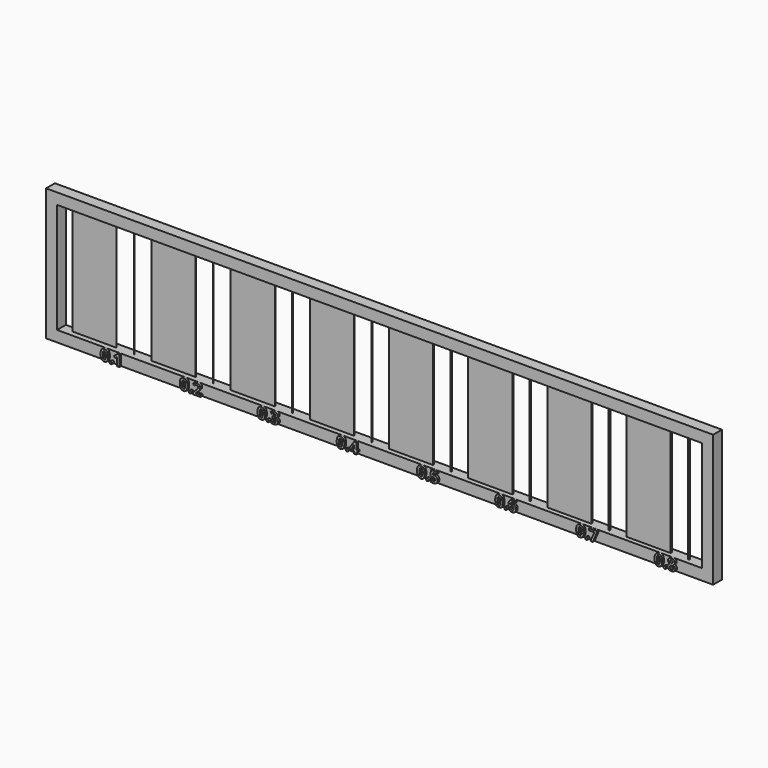
from build123d import *

# Parameters (mm, degrees)
F0_W          = 20
F0_H          = 0.1
F1_DEPTH      = 50
F0_H_2        = 0.2
F0_H_3        = 0.5
F0_H_4        = 0.6
F0_H_5        = 0.7
F0_H_6        = 0.8
F0_H_7        = 0.3
F0_H_8        = 0.4
F0_R          = 0.05
F0_R_2        = 0.1
F0_R_3        = 0.15
F0_R_4        = 0.2
F0_R_5        = 0.25
F0_R_6        = 0.3
F0_R_7        = 0.35
F0_R_8        = 0.4
F2_W          = 303
F2_H          = 60
F2_W_2        = 293
F2_H_2        = 50
F3_DEPTH      = 2.5
F3_DEPTH_BACK = 2.5
F4_TEXT_SIZE  = 6.9444444444
F5_DEPTH      = 1


# Not quite as in the source:
# - Text() gives the source's letters only with a copy of the font that has no kerning and outlines rounded to 1/6400 em; it was checked with that copy


with BuildPart() as f1:
    # F0 (on Top) → F1 (new body)
    with BuildSketch(Plane.XY):
        with Locations((-84.2978805304, 0)):
            Rectangle(F0_W, F0_H)
    extrude(amount=F1_DEPTH)


with BuildPart() as f1b:
    # F0 (on Top) → F1, piece 2 (new body)
    with BuildSketch(Plane.XY):
        with Locations((-48.2978805304, 0)):
            Rectangle(F0_W, F0_H_2)
    extrude(amount=F1_DEPTH)


with BuildPart() as f1c:
    # F0 (on Top) → F1, piece 3 (new body)
    with BuildSketch(Plane.XY):
        with Locations((59.7021194696, 0)):
            Rectangle(F0_W, F0_H_3)
    extrude(amount=F1_DEPTH)


with BuildPart() as f1d:
    # F0 (on Top) → F1, piece 4 (new body)
    with BuildSketch(Plane.XY):
        with Locations((95.7021194696, 0)):
            Rectangle(F0_W, F0_H_4)
    extrude(amount=F1_DEPTH)


with BuildPart() as f1e:
    # F0 (on Top) → F1, piece 5 (new body)
    with BuildSketch(Plane.XY):
        with Locations((131.7021194696, 0)):
            Rectangle(F0_W, F0_H_5)
    extrude(amount=F1_DEPTH)


with BuildPart() as f1f:
    # F0 (on Top) → F1, piece 6 (new body)
    with BuildSketch(Plane.XY):
        with Locations((167.7021194696, 0)):
            Rectangle(F0_W, F0_H_6)
    extrude(amount=F1_DEPTH)


with BuildPart() as f1g:
    # F0 (on Top) → F1, piece 7 (new body)
    with BuildSketch(Plane.XY):
        with Locations((-12.2978805304, 0)):
            Rectangle(F0_W, F0_H_7)
    extrude(amount=F1_DEPTH)


with BuildPart() as f1h:
    # F0 (on Top) → F1, piece 8 (new body)
    with BuildSketch(Plane.XY):
        with Locations((23.7021194696, 0)):
            Rectangle(F0_W, F0_H_8)
    extrude(amount=F1_DEPTH)


with BuildPart() as f1i:
    # F0 (on Top) → F1, piece 9 (new body)
    with BuildSketch(Plane.XY):
        with Locations((-66.2978805304, 0)):
            Circle(F0_R)
    extrude(amount=F1_DEPTH)


with BuildPart() as f1j:
    # F0 (on Top) → F1, piece 10 (new body)
    with BuildSketch(Plane.XY):
        with Locations((-30.2978805304, 0)):
            Circle(F0_R_2)
    extrude(amount=F1_DEPTH)


with BuildPart() as f1k:
    # F0 (on Top) → F1, piece 11 (new body)
    with BuildSketch(Plane.XY):
        with Locations((5.7021194696, 0)):
            Circle(F0_R_3)
    extrude(amount=F1_DEPTH)


with BuildPart() as f1l:
    # F0 (on Top) → F1, piece 12 (new body)
    with BuildSketch(Plane.XY):
        with Locations((41.7021194696, 0)):
            Circle(F0_R_4)
    extrude(amount=F1_DEPTH)


with BuildPart() as f1m:
    # F0 (on Top) → F1, piece 13 (new body)
    with BuildSketch(Plane.XY):
        with Locations((77.7021194696, 0)):
            Circle(F0_R_5)
    extrude(amount=F1_DEPTH)


with BuildPart() as f1n:
    # F0 (on Top) → F1, piece 14 (new body)
    with BuildSketch(Plane.XY):
        with Locations((113.7021194696, 0)):
            Circle(F0_R_6)
    extrude(amount=F1_DEPTH)


with BuildPart() as f1o:
    # F0 (on Top) → F1, piece 15 (new body)
    with BuildSketch(Plane.XY):
        with Locations((149.7021194696, 0)):
            Circle(F0_R_7)
    extrude(amount=F1_DEPTH)


with BuildPart() as f1p:
    # F0 (on Top) → F1, piece 16 (new body)
    with BuildSketch(Plane.XY):
        with Locations((185.7021194696, 0)):
            Circle(F0_R_8)
    extrude(amount=F1_DEPTH)


with BuildPart() as f3:
    # F2 (on Front) → F3 (new body, two sides)
    with BuildSketch(Plane.XZ) as f3_sk:
        with Locations((47.2021194696, 25)):
            Rectangle(F2_W, F2_H)
        with Locations((47.2021194696, 25)):
            Rectangle(F2_W_2, F2_H_2, mode=Mode.SUBTRACT)
    extrude(amount=F3_DEPTH)
    extrude(f3_sk.sketch, amount=-F3_DEPTH_BACK)

    # F4 (on face) → F5 (join)
    with BuildSketch(Plane.XZ.offset(2.5)):
        with Locations((-79.0053535465, -5)):
            Text('0.1', F4_TEXT_SIZE, font='Open Sans', font_style=FontStyle.BOLD, text_align=(TextAlign.LEFT, TextAlign.BOTTOM))
        with Locations((-43.0058725178, -5)):
            Text('0.2', F4_TEXT_SIZE, font='Open Sans', font_style=FontStyle.BOLD, text_align=(TextAlign.LEFT, TextAlign.BOTTOM))
        with Locations((-7.7088745311, -5)):
            Text('0.3', F4_TEXT_SIZE, font='Open Sans', font_style=FontStyle.BOLD, text_align=(TextAlign.LEFT, TextAlign.BOTTOM))
        with Locations((28.2676545903, -5)):
            Text('0.4', F4_TEXT_SIZE, font='Open Sans', font_style=FontStyle.BOLD, text_align=(TextAlign.LEFT, TextAlign.BOTTOM))
        with Locations((64.7441307083, -5)):
            Text('0.5', F4_TEXT_SIZE, font='Open Sans', font_style=FontStyle.BOLD, text_align=(TextAlign.LEFT, TextAlign.BOTTOM))
        with Locations((100.2643853426, -5)):
            Text('0.6', F4_TEXT_SIZE, font='Open Sans', font_style=FontStyle.BOLD, text_align=(TextAlign.LEFT, TextAlign.BOTTOM))
        with Locations((137.027233839, -5)):
            Text('0.7', F4_TEXT_SIZE, font='Open Sans', font_style=FontStyle.BOLD, text_align=(TextAlign.LEFT, TextAlign.BOTTOM))
        with Locations((172.6494170725, -5)):
            Text('0.8', F4_TEXT_SIZE, font='Open Sans', font_style=FontStyle.BOLD, text_align=(TextAlign.LEFT, TextAlign.BOTTOM))
    extrude(amount=F5_DEPTH)


solid = Compound([f1.part, f1b.part, f1c.part, f1d.part, f1e.part, f1f.part, f1g.part, f1h.part, f1i.part, f1j.part, f1k.part, f1l.part, f1m.part, f1n.part, f1o.part, f1p.part, f3.part])
